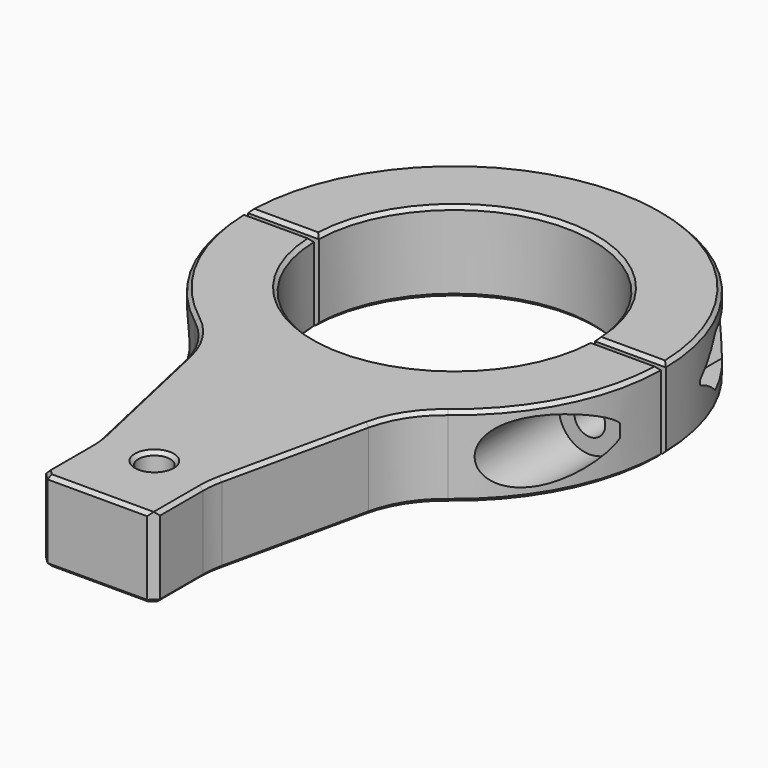
from build123d import *

# Parameters (mm, degrees)
F0_R       = 3.35
F1_DEPTH   = 17
F2_R       = 7.2
F3_DEPTH   = 7
F4_R       = 20
F6_R       = 3.25
F7_DEPTH   = 100
F9_DEPTH   = 38.5
F11_R      = 6.5
F12_DEPTH  = 30
F13_SIZE   = 1.5
F14_SIZE   = 0.74999
F14_2_SIZE = 0.74999


# Not quite as in the source:
# - a fillet or chamfer is up to 0.001 mm smaller than in the source, because OpenCascade refuses the exact size


with BuildPart() as f1:
    # F0 (on Top) → F1 (new body)
    with BuildSketch(Plane.XY):
        with BuildLine():
            ThreePointArc((29.0929715762, -0.6395348837), (0, -29.1), (-29.0929715762, -0.6395348837))
            Line((-29.0929715762, -0.6395348837), (-43.9953519719, -0.6395348837))
            ThreePointArc((-43.9953519719, -0.6395348837), (-37.6443034661, -22.7795174785), (-20.9777310227, -38.6773163643))
            Line((-20.9777310227, -38.6773163643), (-12, -79))
            Line((-12, -79), (-12, -94))
            Line((-12, -94), (12, -94))
            Line((12, -94), (12, -79))
            Line((12, -79), (20.9777310227, -38.6773163643))
            ThreePointArc((20.9777310227, -38.6773163643), (37.6443034661, -22.7795174785), (43.9953519719, -0.6395348837))
            Line((43.9953519719, -0.6395348837), (29.0929715762, -0.6395348837))
        make_face()
        with Locations((0, -79)):
            Circle(F0_R, mode=Mode.SUBTRACT)
    extrude(amount=F1_DEPTH)

    # F2 (on face) → F3 (cut)
    with BuildSketch(Plane(origin=(0, 0, 0), x_dir=(1, 0, 0), z_dir=(0, 0, -1))):
        with Locations((0, 79)):
            Circle(F2_R)
    extrude(amount=-F3_DEPTH, mode=Mode.SUBTRACT)

    # F4
    f4_edges = [f1.edges().sort_by_distance(p)[0] for p in [
        (-20.977731, -38.677316, 8.5),
        (-12, -79, 8.5),
        (20.977731, -38.677316, 8.5),
        (12, -79, 8.5),
    ]]
    fillet(f4_edges, radius=F4_R)


with BuildPart() as f1b:
    # F0 (on Top) → F1, piece 2 (new body)
    with BuildSketch(Plane.XY):
        with BuildLine():
            ThreePointArc((43.9953519719, 0.6395348837), (0, 44), (-43.9953519719, 0.6395348837))
            Line((-43.9953519719, 0.6395348837), (-29.0929715762, 0.6395348837))
            ThreePointArc((-29.0929715762, 0.6395348837), (0, 29.1), (29.0929715762, 0.6395348837))
            Line((29.0929715762, 0.6395348837), (43.9953519719, 0.6395348837))
        make_face()
    extrude(amount=F1_DEPTH)


with BuildPart() as f7_tool:
    # F6 (on offset) → F7 (new body)
    with BuildSketch(Plane.XZ.offset(-50)):
        with Locations((36.4953519719, 8.5)):
            Circle(F6_R)
        with Locations((-36.4953519719, 8.5)):
            Circle(F6_R)
    extrude(amount=F7_DEPTH)


with BuildPart() as f1_1:
    add(f1.part)

    # F7: cut by f7_tool
    add(f7_tool.part, mode=Mode.SUBTRACT)

    # F11 (on offset) → F12 (cut)
    with BuildSketch(Plane.XZ.offset(40)):
        with Locations((-36.4953519719, 8.5)):
            Circle(F11_R)
        with Locations((36.4953519719, 8.5)):
            Circle(F11_R)
    extrude(amount=-F12_DEPTH, mode=Mode.SUBTRACT)

    # F13
    f13_edges = [f1_1.edges().sort_by_distance(p)[0] for p in [
        (-12, -94, 8.5),
        (12, -94, 8.5),
    ]]
    chamfer(f13_edges, length=F13_SIZE)

    # F14 (size 0.75 in the source; OpenCascade refuses exactly that, so slightly less here)
    f14_edges = [f1_1.edges().sort_by_distance(p)[0] for p in [
        (-3.35, -79, 17),
        (0, -29.1, 17),
        (36.544162, -0.639535, 17),
        (-36.544162, -0.639535, 17),
        (-7.2, -79, 0),
        (0, -29.1, 0),
        (39.276157, -19.833898, 0),
        (21.89664, -40.155533, 0),
        (15.8459, -61.726481, 0),
        (12, -86.849771, 0),
        (12.119863, -79.013182, 0),
        (11.25, -93.25, 0),
        (0, -94, 0),
        (-11.25, -93.25, 0),
        (-12, -86.849771, 0),
        (-12.119863, -79.013182, 0),
        (-15.8459, -61.726481, 0),
        (-21.89664, -40.155533, 0),
        (-39.276157, -19.833898, 0),
        (15.8459, -61.726481, 17),
        (21.89664, -40.155533, 17),
        (39.276157, -19.833898, 17),
        (-15.8459, -61.726481, 17),
        (-12, -86.849771, 17),
        (-12.119863, -79.013182, 17),
        (-11.25, -93.25, 17),
        (0, -94, 17),
        (12, -86.849771, 17),
        (-39.276157, -19.833898, 17),
        (-21.89664, -40.155533, 17),
    ]]
    chamfer(f14_edges, length=F14_SIZE)


with BuildPart() as f1b_1:
    add(f1b.part)

    # F7: cut by f7_tool
    add(f7_tool.part, mode=Mode.SUBTRACT)

    # F8 (on offset) → F9 (cut)
    with BuildSketch(Plane.XZ.offset(-50)):
        Polygon((30.2599690647, 8.5), (33.3776605183, 3.1), (39.6130434255, 3.1), (42.7307348792, 8.5), (39.6130434255, 13.9), (33.3776605183, 13.9), align=None)
        Polygon((-42.7307348792, 8.5), (-39.6130434255, 3.1), (-33.3776605183, 3.1), (-30.2599690647, 8.5), (-33.3776605183, 13.9), (-39.6130434255, 13.9), align=None)
    extrude(amount=F9_DEPTH, mode=Mode.SUBTRACT)

    # F14#2 (size 0.75 in the source; OpenCascade refuses exactly that, so slightly less here)
    f14_2_edges = [f1b_1.edges().sort_by_distance(p)[0] for p in [
        (0, 29.1, 17),
        (36.544162, 0.639535, 17),
        (-36.544162, 0.639535, 17),
        (0, 29.1, 0),
        (0, 44, 0),
        (0, 44, 17),
    ]]
    chamfer(f14_2_edges, length=F14_2_SIZE)


solid = Compound([f1_1.part, f1b_1.part])
